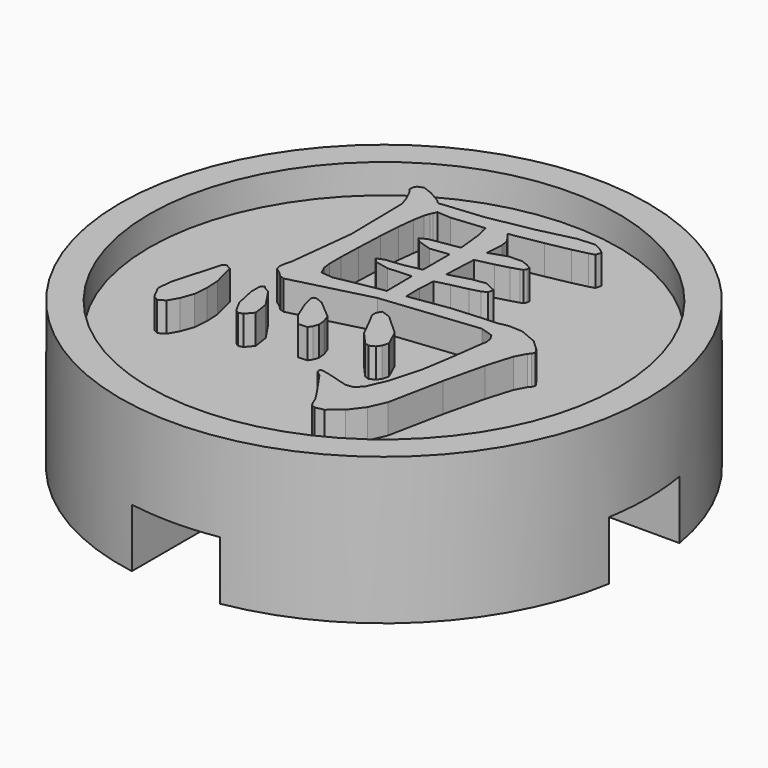
from build123d import *

# Parameters (mm, degrees)
F0_R     = 9
F1_DEPTH = 4
F3_W     = 3
F3_H     = 3
F4_DEPTH = 2
F2_R     = 9
F2_R_2   = 8
F5_DEPTH = 1
F7_DEPTH = 1


# Not quite as in the source:
# - a feature names something its author has since deleted; it is built from what else it names


with BuildPart() as f1:
    # F0 (on Top) → F1 (new body)
    with BuildSketch(Plane.XY):
        with Locations((-31.3306450844, 19.7580661625)):
            Circle(F0_R)
    extrude(amount=F1_DEPTH)

    # F3 (on face) → F4 (cut)
    with BuildSketch(Plane(origin=(0, 0, 0), x_dir=(1, 0, 0), z_dir=(0, 0, -1))):
        with BuildLine():
            ThreePointArc((-32.8306450844, -28.6321858371), (-32.0832814269, -28.7265408676), (-31.3306450844, -28.7580661625))
            ThreePointArc((-31.3306450844, -28.7580661625), (-30.5780087419, -28.7265408676), (-29.8306450844, -28.6321858371))
            Line((-29.8306450844, -28.6321858371), (-29.8306450844, -21.2580661625))
            Line((-29.8306450844, -21.2580661625), (-32.8306450844, -21.2580661625))
            Line((-32.8306450844, -21.2580661625), (-32.8306450844, -28.6321858371))
        make_face()
        with BuildLine():
            ThreePointArc((-40.204764759, -18.2580661625), (-40.2991197895, -19.0054298199), (-40.3306450844, -19.7580661625))
            ThreePointArc((-40.3306450844, -19.7580661625), (-40.2991197895, -20.510702505), (-40.204764759, -21.2580661625))
            Line((-40.204764759, -21.2580661625), (-32.8306450844, -21.2580661625))
            Line((-32.8306450844, -21.2580661625), (-32.8306450844, -18.2580661625))
            Line((-32.8306450844, -18.2580661625), (-40.204764759, -18.2580661625))
        make_face()
        with Locations((-31.3306450844, -19.7580661625)):
            Rectangle(F3_W, F3_H)
        with BuildLine():
            Line((-29.8306450844, -18.2580661625), (-29.8306450844, -21.2580661625))
            Line((-29.8306450844, -21.2580661625), (-22.4565254097, -21.2580661625))
            ThreePointArc((-22.4565254097, -21.2580661625), (-22.3621703793, -20.510702505), (-22.3306450844, -19.7580661625))
            ThreePointArc((-22.3306450844, -19.7580661625), (-22.3621703793, -19.0054298199), (-22.4565254097, -18.2580661625))
            Line((-22.4565254097, -18.2580661625), (-29.8306450844, -18.2580661625))
        make_face()
        with BuildLine():
            Line((-32.8306450844, -10.8839464878), (-32.8306450844, -18.2580661625))
            Line((-32.8306450844, -18.2580661625), (-29.8306450844, -18.2580661625))
            Line((-29.8306450844, -18.2580661625), (-29.8306450844, -10.8839464878))
            ThreePointArc((-29.8306450844, -10.8839464878), (-30.5780087419, -10.7895914574), (-31.3306450844, -10.7580661625))
            ThreePointArc((-31.3306450844, -10.7580661625), (-32.0832814269, -10.7895914574), (-32.8306450844, -10.8839464878))
        make_face()
    extrude(amount=-F4_DEPTH, mode=Mode.SUBTRACT)

    # F2 (on face) → F5 (join)
    with BuildSketch(Plane.XY.offset(4)):
        with Locations((-31.3306450844, 19.7580661625)):
            Circle(F2_R)
        with Locations((-31.3306450844, 19.7580661625)):
            Circle(F2_R_2, mode=Mode.SUBTRACT)
    extrude(amount=F5_DEPTH)

    # F6 (on face) → F7 (join)
    with BuildSketch(Plane.XY.offset(4)):
        Polygon((-30.2867247296, 22.1786791809), (-30.9853611304, 21.9775667851), (-30.9337890524, 23.0947539388), (-30.3425373169, 23.2288288693), (-29.9085710651, 23.346503006), (-29.6396105184, 23.4307519507), (-29.5382124546, 23.4659855953), (-29.4952461164, 23.5484884479), (-29.4832105529, 23.6550624275), (-29.6542028597, 23.7521576214), (-29.8853729841, 23.8406470756), (-30.3451564551, 23.8217518644), (-30.920038577, 23.6275614767), (-30.8787933868, 24.2256603877), (-30.9174693272, 24.4877612868), (-31.1606687791, 24.8134698273), (-31.1709644865, 24.8271891225), (-30.0735767703, 25.0179496865), (-29.2761115556, 25.1778418362), (-28.7811568004, 25.2920861491), (-28.5929530142, 25.3462773652), (-28.5379511125, 25.5455813084), (-28.689175162, 25.6625071199), (-28.9641846707, 25.8000118743), (-29.5511210642, 25.7570455361), (-30.7206847454, 25.4802899353), (-32.2253983367, 25.1992938251), (-33.5977830895, 25.0643458485), (-33.6630994069, 25.0403370819), (-33.7516013331, 25.0755707264), (-33.8108936326, 25.1468487011), (-34.2526175223, 25.4029629986), (-34.570562189, 25.5180803576), (-34.7501727076, 25.4493591606), (-34.8077500952, 25.3599966604), (-34.8232154825, 25.2061534727), (-34.714939063, 25.0781275041), (-34.5447886221, 24.7171853191), (-34.450256442, 24.4387459866), (-34.4124473116, 22.2354271747), (-34.6633794572, 19.9804739245), (-34.738997718, 19.6960168103), (-34.7424337778, 19.5817288451), (-34.7089212813, 19.4193110979), (-34.5293169987, 19.2895328012), (-34.3720502232, 19.1382900435), (-34.2233829514, 19.0901727335), (-31.5697033299, 19.7716288351), (-28.2870127309, 20.1282681503), (-27.8607791726, 19.9941932198), (-27.7430426755, 19.8120196874), (-27.7129225865, 19.609229796), (-27.7585080628, 19.3445347029), (-27.8186858805, 18.8830737362), (-27.9131619362, 18.2041744124), (-28.0601454763, 17.2889789366), (-28.3514310579, 16.2362599983), (-28.6307434365, 15.597770235), (-28.8387154799, 15.3657520087), (-29.1119788964, 15.33309385), (-29.8578720332, 15.5462106291), (-30.0649710305, 15.5883163934), (-30.1638123165, 15.5840197595), (-30.1681151864, 15.4637140126), (-29.9919469637, 15.33309385), (-29.6498999898, 14.8372473407), (-29.3834962208, 14.4505378248), (-29.2056442665, 14.16265837), (-29.1256981916, 13.9615696711), (-29.0621529106, 13.8472754699), (-28.926331888, 13.8000118743), (-28.636730038, 13.8627439753), (-28.2045098783, 14.2124999459), (-27.8453137853, 14.6885800689), (-27.5926293116, 15.2540332933), (-27.2154110535, 17.1385905168), (-26.889702513, 18.5178411533), (-26.6267285679, 19.390949573), (-26.4342219118, 19.7535879619), (-26.3577680212, 19.8335090926), (-26.3139286369, 19.9529667376), (-26.4282353103, 20.1196624106), (-26.767663146, 20.4342084336), (-27.3563456317, 20.6808439454), (-27.8194965661, 20.6988661105), (-28.1581137162, 20.635258469), (-28.4863790345, 20.6197930817), (-29.6722873852, 20.5321766736), (-31.0266063206, 20.327634454), (-31.0369269723, 20.90340833), (-30.9991053698, 21.4585409029), (-30.5255901314, 21.5762774), (-29.9782276685, 21.6991898131), (-29.6516460819, 21.790236045), (-29.4832105529, 21.8710551659), (-29.431638475, 22.0600696377), (-29.8303710823, 22.2457166462), align=None)
        Polygon((-31.6384557071, 22.9331780574), (-31.6384557071, 21.8057014323), (-32.2099329494, 21.6871542495), (-32.796875579, 21.6201167843), (-33.0331904391, 21.529881238), (-32.9034183784, 21.3794678741), (-32.4282069363, 21.2806265881), (-31.6797008974, 21.3279581566), (-31.6874460631, 21.3073168533), (-31.6384557071, 21.3279581566), (-31.6247052317, 20.2485614252), (-32.5218847784, 20.0913507741), (-33.250610088, 19.9529667376), (-33.6467547374, 19.990763396), (-33.7696422063, 20.2623430808), (-33.8005979252, 20.5210141561), (-33.8014522631, 21.0142851796), (-33.779102284, 21.7223255336), (-33.7421412554, 22.6272377741), (-33.6948907555, 23.3396433584), (-33.6321499241, 23.8887893297), (-33.565137403, 24.2591479401), (-33.5049658214, 24.4387459866), (-33.4697446489, 24.5100863217), (-33.4087187294, 24.6381122903), (-32.9369433471, 24.6071815156), (-31.9443959904, 24.7068958476), (-31.8378344829, 24.7206151429), (-31.7261220035, 24.2720565497), (-31.6384557071, 23.428195173), (-32.6387419934, 23.2666192916), (-32.8656217201, 23.1488827945), (-32.7453097371, 23.01568091), (-32.2640742771, 22.8627107683), (-31.6934513728, 22.9331780574), align=None, mode=Mode.SUBTRACT)
        Polygon((-35.9936497153, 18.6716593969), (-36.021149419, 18.5676920833), (-36.4473873424, 17.0518035025), (-36.486058294, 16.5653921266), (-36.261767149, 16.1305777729), (-36.0821641137, 16.0274460891), (-35.8595897513, 16.1580787237), (-35.6722527751, 16.487210852), (-35.5158528097, 16.917734808), (-35.4788980172, 17.4041212397), (-35.5021023342, 17.8767759041), (-35.7014748739, 18.6501886999), (-35.8080301455, 18.7034694537), (-35.8733402267, 18.7430059681), align=None)
        Polygon((-34.4227554912, 18.3030156984), (-34.4227554912, 17.9558239887), (-34.2775180432, 17.2752284612), (-34.0618382503, 16.8764896178), (-33.9337811015, 16.7922718533), (-33.7833926817, 16.8386680153), (-33.5702821387, 17.0895939248), (-33.6493489314, 17.612080811), (-34.0377733592, 18.1964479548), (-34.0755887257, 18.2480200327), (-34.2302675432, 18.333946473), (-34.3161939836, 18.4095584978), (-34.3935458644, 18.3760522373), align=None)
        Polygon((-32.9309193293, 18.6089372736), (-32.8381207692, 18.2617642721), (-32.5949213173, 17.6670764767), (-32.2778185165, 17.278658285), (-31.9718969413, 17.302723176), (-31.8902608987, 17.4264712188), (-31.8240840074, 17.6086509872), (-31.8532998702, 17.8604561788), (-31.9443959904, 18.117387398), (-32.5562453769, 18.6364382244), (-32.7324135996, 18.7086204254), (-32.8381207692, 18.7430059681), (-32.9180231918, 18.7163593551), align=None)
        Polygon((-31.0609669191, 18.9011146094), (-30.9475395279, 18.7017545418), (-30.5771622093, 17.9661384043), (-30.1913132674, 17.5295841945), (-30.0383431257, 17.4797519726), (-29.8578720332, 17.5708293847), (-29.7556009234, 17.708327903), (-29.6962961518, 17.9283230379), (-29.9567133192, 18.4963704563), (-30.6381881289, 19.1142438606), (-30.6519386043, 19.127994336), (-30.8349727106, 19.1941462831), (-30.9716106549, 19.2345371355), (-31.0644216871, 19.0764284941), align=None)
    extrude(amount=F7_DEPTH)


solid = f1.part
